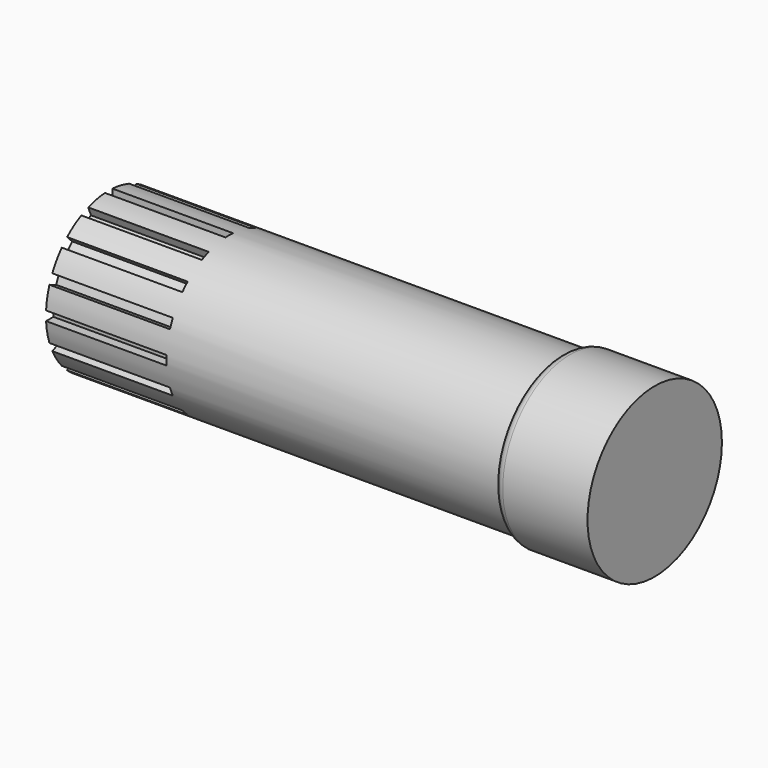
from build123d import *

# Parameters (mm, degrees)
F0_R     = 9
F1_DEPTH = 10
F2_R     = 8.4
F3_DEPTH = 48.5
F6_DEPTH = 12.919


# Not quite as in the source:
# - a fillet or chamfer that OpenCascade refuses, or shapes differently, is made with other operations: its cross-section is extruded or revolved along the edge and cut away or added


with BuildPart() as f1:
    # F0 (on Right) → F1 (new body)
    with BuildSketch(Plane.YZ):
        Circle(F0_R)
    extrude(amount=F1_DEPTH)

    # F2 (on Right) → F3 (join)
    with BuildSketch(Plane.YZ):
        Circle(F2_R)
    extrude(amount=-F3_DEPTH)

    # F4: fillet of radius 1 on 1 edges, made by hand

    # F4_s1 → F4_t2 (revolve, cut)
    with BuildSketch(Plane.XY):
        with BuildLine():
            ThreePointArc((0.916515139, 9), (0.3687925815, 8.8366600265), (0, 8.4))
            Line((0, 8.4), (0, 9))
            Line((0, 9), (0.916515139, 9))
        make_face()
    revolve(axis=Axis((0, 0, 0), (1, 0, 0)), mode=Mode.SUBTRACT)

    # F5 (on face) → F6 (cut)
    with BuildSketch(Plane(origin=(-48.5, 0, 0), x_dir=(0, -1, 0), z_dir=(-1, 0, 0))):
        with BuildLine():
            Line((0.5, 7.4), (0.5, 8.3851058431))
            ThreePointArc((0.5, 8.3851058431), (0, 8.4), (-0.5, 8.3851058431))
            Line((-0.5, 8.3851058431), (-0.5, 7.4))
            Line((-0.5, 7.4), (0.5, 7.4))
        make_face()
        with BuildLine():
            Line((-2.3699176332, 7.0280502568), (-2.7469013185, 7.9381693826))
            ThreePointArc((-2.7469013185, 7.9381693826), (-3.2145408319, 7.7605880731), (-3.670780851, 7.5554859502))
            Line((-3.670780851, 7.5554859502), (-3.2937971658, 6.6453668244))
            Line((-3.2937971658, 6.6453668244), (-2.3699176332, 7.0280502568))
        make_face()
        with BuildLine():
            Line((-4.8790367902, 5.5861435714), (-5.575611812, 6.2827185932))
            ThreePointArc((-5.575611812, 6.2827185932), (-5.939696962, 5.939696962), (-6.2827185932, 5.575611812))
            Line((-6.2827185932, 5.575611812), (-5.5861435714, 4.8790367902))
            Line((-5.5861435714, 4.8790367902), (-4.8790367902, 5.5861435714))
        make_face()
        with BuildLine():
            Line((-6.6453668244, 3.2937971658), (-7.5554859502, 3.670780851))
            ThreePointArc((-7.5554859502, 3.670780851), (-7.7605880731, 3.2145408319), (-7.9381693826, 2.7469013185))
            Line((-7.9381693826, 2.7469013185), (-7.0280502568, 2.3699176332))
            Line((-7.0280502568, 2.3699176332), (-6.6453668244, 3.2937971658))
        make_face()
        with BuildLine():
            Line((-7.4, 0.5), (-8.3851058431, 0.5))
            ThreePointArc((-8.3851058431, 0.5), (-8.4, 0), (-8.3851058431, -0.5))
            Line((-8.3851058431, -0.5), (-7.4, -0.5))
            Line((-7.4, -0.5), (-7.4, 0.5))
        make_face()
        with BuildLine():
            Line((-7.0280502568, -2.3699176332), (-7.9381693826, -2.7469013185))
            ThreePointArc((-7.9381693826, -2.7469013185), (-7.7605880731, -3.2145408319), (-7.5554859502, -3.670780851))
            Line((-7.5554859502, -3.670780851), (-6.6453668244, -3.2937971658))
            Line((-6.6453668244, -3.2937971658), (-7.0280502568, -2.3699176332))
        make_face()
        with BuildLine():
            Line((-5.5861435714, -4.8790367902), (-6.2827185932, -5.575611812))
            ThreePointArc((-6.2827185932, -5.575611812), (-5.939696962, -5.939696962), (-5.575611812, -6.2827185932))
            Line((-5.575611812, -6.2827185932), (-4.8790367902, -5.5861435714))
            Line((-4.8790367902, -5.5861435714), (-5.5861435714, -4.8790367902))
        make_face()
        with BuildLine():
            Line((-3.2937971658, -6.6453668244), (-3.670780851, -7.5554859502))
            ThreePointArc((-3.670780851, -7.5554859502), (-3.2145408319, -7.7605880731), (-2.7469013185, -7.9381693826))
            Line((-2.7469013185, -7.9381693826), (-2.3699176332, -7.0280502568))
            Line((-2.3699176332, -7.0280502568), (-3.2937971658, -6.6453668244))
        make_face()
        with BuildLine():
            Line((-0.5, -7.4), (-0.5, -8.3851058431))
            ThreePointArc((-0.5, -8.3851058431), (0, -8.4), (0.5, -8.3851058431))
            Line((0.5, -8.3851058431), (0.5, -7.4))
            Line((0.5, -7.4), (-0.5, -7.4))
        make_face()
        with BuildLine():
            Line((2.3699176332, -7.0280502568), (2.7469013185, -7.9381693826))
            ThreePointArc((2.7469013185, -7.9381693826), (3.2145408319, -7.7605880731), (3.670780851, -7.5554859502))
            Line((3.670780851, -7.5554859502), (3.2937971658, -6.6453668244))
            Line((3.2937971658, -6.6453668244), (2.3699176332, -7.0280502568))
        make_face()
        with BuildLine():
            Line((4.8790367902, -5.5861435714), (5.575611812, -6.2827185932))
            ThreePointArc((5.575611812, -6.2827185932), (5.939696962, -5.939696962), (6.2827185932, -5.575611812))
            Line((6.2827185932, -5.575611812), (5.5861435714, -4.8790367902))
            Line((5.5861435714, -4.8790367902), (4.8790367902, -5.5861435714))
        make_face()
        with BuildLine():
            Line((6.6453668244, -3.2937971658), (7.5554859502, -3.670780851))
            ThreePointArc((7.5554859502, -3.670780851), (7.7605880731, -3.2145408319), (7.9381693826, -2.7469013185))
            Line((7.9381693826, -2.7469013185), (7.0280502568, -2.3699176332))
            Line((7.0280502568, -2.3699176332), (6.6453668244, -3.2937971658))
        make_face()
        with BuildLine():
            Line((7.4, -0.5), (8.3851058431, -0.5))
            ThreePointArc((8.3851058431, -0.5), (8.4, 0), (8.3851058431, 0.5))
            Line((8.3851058431, 0.5), (7.4, 0.5))
            Line((7.4, 0.5), (7.4, -0.5))
        make_face()
        with BuildLine():
            Line((7.0280502568, 2.3699176332), (7.9381693826, 2.7469013185))
            ThreePointArc((7.9381693826, 2.7469013185), (7.7605880731, 3.2145408319), (7.5554859502, 3.670780851))
            Line((7.5554859502, 3.670780851), (6.6453668244, 3.2937971658))
            Line((6.6453668244, 3.2937971658), (7.0280502568, 2.3699176332))
        make_face()
        with BuildLine():
            Line((5.5861435714, 4.8790367902), (6.2827185932, 5.575611812))
            ThreePointArc((6.2827185932, 5.575611812), (5.939696962, 5.939696962), (5.575611812, 6.2827185932))
            Line((5.575611812, 6.2827185932), (4.8790367902, 5.5861435714))
            Line((4.8790367902, 5.5861435714), (5.5861435714, 4.8790367902))
        make_face()
        with BuildLine():
            Line((3.2937971658, 6.6453668244), (3.670780851, 7.5554859502))
            ThreePointArc((3.670780851, 7.5554859502), (3.2145408319, 7.7605880731), (2.7469013185, 7.9381693826))
            Line((2.7469013185, 7.9381693826), (2.3699176332, 7.0280502568))
            Line((2.3699176332, 7.0280502568), (3.2937971658, 6.6453668244))
        make_face()
    extrude(amount=-F6_DEPTH, mode=Mode.SUBTRACT)


solid = f1.part
